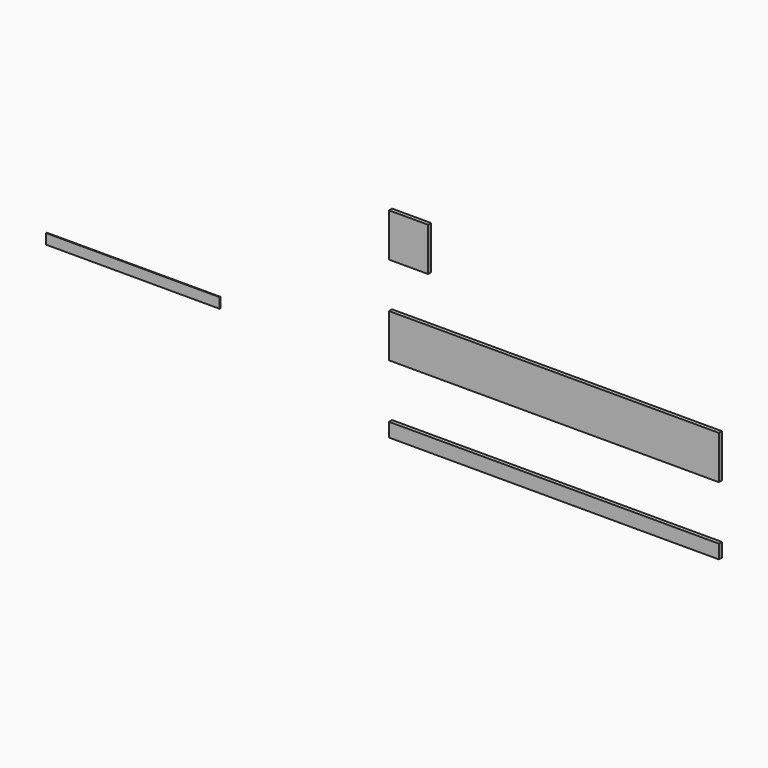
from build123d import *

# Parameters (mm, degrees)
F0_W     = 57.15
F0_H     = 63.5
F1_DEPTH = 5.588
F0_W_2   = 482.6
F0_H_2   = 20.32
F2_W     = 254
F2_H     = 15
F3_DEPTH = 1.27


# Not quite as in the source:
# - a feature names something its author has since deleted; it is built from what else it names


with BuildPart() as f1:
    # F0 (on Front) → F1 (new body)
    with BuildSketch(Plane.XZ):
        with Locations((28.575, 31.75)):
            Rectangle(F0_W, F0_H)
    extrude(amount=F1_DEPTH)


with BuildPart() as f1b:
    # F0 (on Front) → F1, piece 2 (new body)
    with BuildSketch(Plane.XZ):
        with Locations((241.3, -97.9633150748)):
            Rectangle(F0_W_2, F0_H)
    extrude(amount=F1_DEPTH)


with BuildPart() as f1c:
    # F0 (on Front) → F1, piece 3 (new body)
    with BuildSketch(Plane.XZ):
        with Locations((241.3, -219.0275779629)):
            Rectangle(F0_W_2, F0_H_2)
    extrude(amount=F1_DEPTH)


with BuildPart() as f3:
    # F2 (on Front) → F3 (new body)
    with BuildSketch(Plane.XZ):
        with Locations((-378.1612176895, -139.3002796173)):
            Rectangle(F2_W, F2_H)
    extrude(amount=F3_DEPTH)


solid = Compound([f1.part, f1b.part, f1c.part, f3.part])
